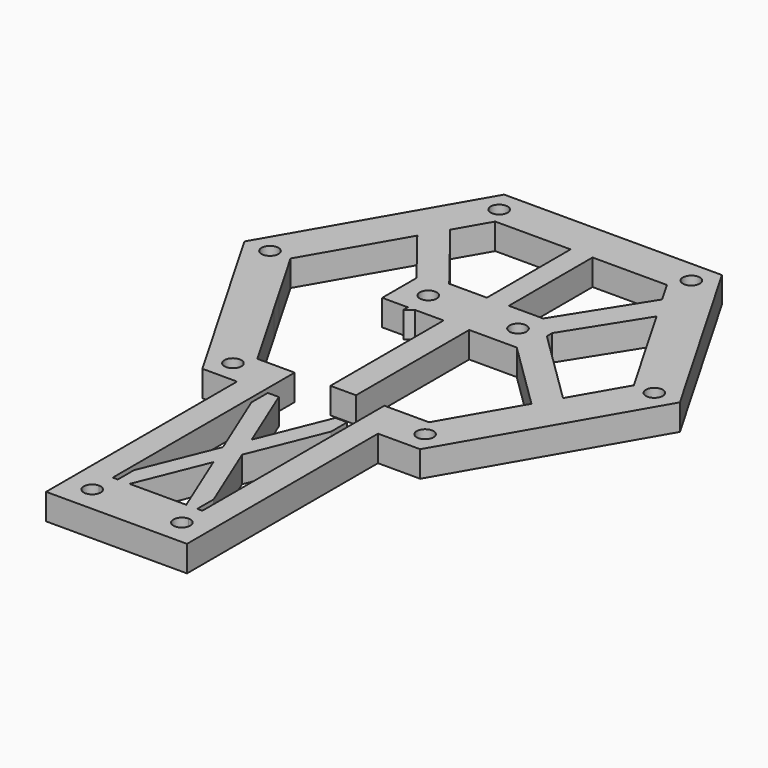
from build123d import *

# Parameters (mm, degrees)
F0_R     = 1.65
F0_W     = 5
F0_H     = 36.5884533238
F0_H_2   = 27.6073180421
F0_W_2   = 4.2823543772
F0_H_3   = 20.4163840114
F1_DEPTH = 5.08


# Not quite as in the source:
# - a feature names something its author has since deleted; it is built from what else it names


with BuildPart() as f1:
    # F0 (on Top) → F1 (new body)
    with BuildSketch(Plane.XY):
        Polygon((21.25, 36.8060796608), (-21.25, 36.8060796608), (-42.5, 0), (-21.25, -36.8060796608), (-14.481, -36.8060796608), (-9.481, -36.8060796608), (-9.481, -29.0118510268), (-16.75, -29.0118510268), (-25.125, -14.5059255134), (-27.6471267629, -10.137473817), (-33.5, 0), (-23.128253194, 17.9643924312), (-20.4351344929, 22.6290108523), (-16.75, 29.0118510268), (-2.0468940441, 29.0118510268), (2.2354603331, 29.0118510268), (16.75, 29.0118510268), (19.1722516141, 24.8163881624), (21.9975489559, 19.92282962), (33.5, 0), (27.7069725582, -10.0338178588), (25.125, -14.5059255134), (16.75, -29.0118510268), (8.019, -29.0118510268), (8.019, -36.8060796608), (13.019, -36.8060796608), (21.25, -36.8060796608), (42.5, 0), align=None)
        with Locations((-18.75, -32.4759526419)):
            Circle(F0_R, mode=Mode.SUBTRACT)
        with Locations((18.75, -32.4759526419)):
            Circle(F0_R, mode=Mode.SUBTRACT)
        with Locations((-37.5, 0)):
            Circle(F0_R, mode=Mode.SUBTRACT)
        with Locations((-18.75, 32.4759526419)):
            Circle(F0_R, mode=Mode.SUBTRACT)
        with Locations((37.5, 0)):
            Circle(F0_R, mode=Mode.SUBTRACT)
        with Locations((18.75, 32.4759526419)):
            Circle(F0_R, mode=Mode.SUBTRACT)
        with Locations((-11.981, -55.1003063227)):
            Rectangle(F0_W, F0_H)
        with Locations((10.519, -55.1003063227)):
            Rectangle(F0_W, F0_H)
        Polygon((-9.481, -73.3945329846), (-14.481, -73.3945329846), (-14.481, -83.3945329846), (13.019, -83.3945329846), (13.019, -73.3945329846), (8.019, -73.3945329846), (7.019, -73.3945329846), (4.8774445356, -73.3945329846), (-6.1735640291, -73.3945329846), (-8.481, -73.3945329846), align=None)
        with BuildLine():
            ThreePointArc((-7.831, -78.3945329846), (-10.647726189, -79.5612591736), (-9.481, -76.7445329846))
            ThreePointArc((-9.481, -76.7445329846), (-8.314273811, -77.2278067957), (-7.831, -78.3945329846))
        make_face(mode=Mode.SUBTRACT)
        with BuildLine():
            ThreePointArc((9.669, -78.3945329846), (6.852273811, -79.5612591736), (8.019, -76.7445329846))
            ThreePointArc((8.019, -76.7445329846), (9.185726189, -77.2278067957), (9.669, -78.3945329846))
        make_face(mode=Mode.SUBTRACT)
        Polygon((-6.3394445356, -36.8060796608), (-8.481, -36.8060796608), (-8.481, -40.8093024077), (-2.6512739295, -55.0297430961), (-0.7737012417, -50.3825876202), align=None)
        Polygon((7.019, -40.7417911932), (7.019, -36.8060796608), (4.7115640291, -36.8060796608), (-0.7737012417, -50.3825876202), (1.1892739295, -55.1708695493), align=None)
        with Locations((-0.002691932, -15.2081920057)):
            Rectangle(F0_W, F0_H_2)
        Polygon((-9.481, -1.4045329846), (-9.481, -2.4605728254), (-8.1094596477, -1.4045329846), align=None)
        Polygon((-8.481, -69.4588214522), (-8.481, -73.3945329846), (-6.1735640291, -73.3945329846), (-0.6882987583, -59.8180250252), (-2.6512739295, -55.0297430961), align=None)
        Polygon((4.8774445356, -73.3945329846), (7.019, -73.3945329846), (7.019, -69.3913102377), (1.1892739295, -55.1708695493), (-0.6882987583, -59.8180250252), align=None)
        Polygon((2.497308068, -1.4045329846), (8.019, -1.4045329846), (11.781800831, -1.4045329846), (13.019, -1.4045329846), (13.019, 4.3879779564), (13.019, 5.6842228109), (13.019, 8.5954670154), (8.9436992999, 8.5954670154), (2.2354603331, 8.5954670154), (-2.0468940441, 8.5954670154), (-9.4036843662, 8.5954670154), (-14.481, 8.5954670154), (-14.481, 6.9638797721), (-14.481, 0), (-14.481, -1.4045329846), (-9.481, -1.4045329846), (-8.1094596477, -1.4045329846), (-2.502691932, -1.4045329846), align=None)
        with BuildLine():
            ThreePointArc((-7.831, 3.5954670154), (-8.314273811, 2.4287408264), (-9.481, 1.9454670154))
            ThreePointArc((-9.481, 1.9454670154), (-10.647726189, 4.7621932043), (-7.831, 3.5954670154))
        make_face(mode=Mode.SUBTRACT)
        with BuildLine():
            ThreePointArc((9.669, 3.5954670154), (9.185726189, 2.4287408264), (8.019, 1.9454670154))
            ThreePointArc((8.019, 1.9454670154), (6.852273811, 4.7621932043), (9.669, 3.5954670154))
        make_face(mode=Mode.SUBTRACT)
        Polygon((1.1892739295, -55.1708695493), (-0.7737012417, -50.3825876202), (-2.6512739295, -55.0297430961), (-0.6882987583, -59.8180250252), align=None)
        Polygon((11.781800831, -1.4045329846), (25.125, -14.5059255134), (27.7069725582, -10.0338178588), (13.019, 4.3879779564), (13.019, -1.4045329846), align=None)
        Polygon((-20.4351344929, 22.6290108523), (-23.128253194, 17.9643924312), (-14.481, 6.9638797721), (-14.481, 8.5954670154), (-9.4036843662, 8.5954670154), align=None)
        Polygon((13.019, 5.6842228109), (21.9975489559, 19.92282962), (19.1722516141, 24.8163881624), (8.9436992999, 8.5954670154), (13.019, 8.5954670154), align=None)
        with Locations((0.0942831445, 18.8036590211)):
            Rectangle(F0_W_2, F0_H_3)
    extrude(amount=F1_DEPTH)


solid = f1.part
